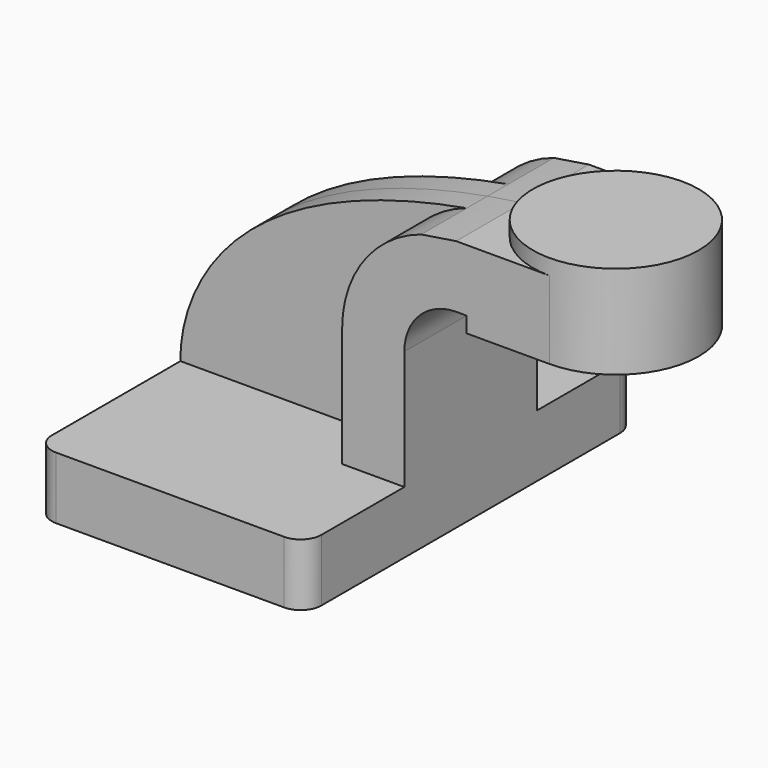
from build123d import *

# Parameters (mm, degrees)
F1_DEPTH = 63.5
F2_DEPTH = 25.4
F3_DEPTH = 7.9375
F5_R     = 6.35


# Not quite as in the source:
# - a feature names something its author has since deleted; it is built from what else it names


with BuildPart() as f1:
    # F0 (on Front) → F1 (new body, symmetric)
    with BuildSketch(Plane.XZ):
        Polygon((41.275, -9.525), (41.275, 9.525), (22.225, 9.525), (-41.275, 9.525), (-41.275, -9.525), align=None)
    extrude(amount=F1_DEPTH, both=True)

    # F0 (on Front) → F2 (join, symmetric)
    with BuildSketch(Plane.XZ):
        with BuildLine():
            Line((22.225, 9.525), (41.275, 9.525))
            Line((41.275, 9.525), (41.275, 46.0502))
            ThreePointArc((41.275, 46.0502), (45.9246798487, 57.2755201513), (57.15, 61.9252))
            Line((57.15, 61.9252), (60.325, 61.9252))
            Line((60.325, 61.9252), (60.325, 80.9752))
            Line((60.325, 80.9752), (57.15, 80.9752))
            add(Edge.make_bspline(
                [(46.42519144, 79.2877406183), (49.8648948299, 79.9027002695), (53.4381248944, 80.4666827005), (57.15, 80.9752)],
                knots=[116.6855453381, 116.6855453381, 116.6855453381, 116.6855453381, 121.6248811101, 121.6248811101, 121.6248811101, 121.6248811101], degree=3))
            ThreePointArc((46.42519144, 79.2877406183), (28.9159818308, 66.6073360608), (22.225, 46.0502))
            Line((22.225, 46.0502), (22.225, 9.525))
        make_face()
        Polygon((60.325, 80.9752), (60.325, 61.9252), (60.325, 57.15), (85.725, 57.15), (85.725, 80.9752), align=None)
    extrude(amount=F2_DEPTH, both=True)

    # F0 (on Front) → F3 (join, symmetric)
    with BuildSketch(Plane.XZ):
        with BuildLine():
            Line((-41.275, 9.525), (22.225, 9.525))
            Line((22.225, 9.525), (22.225, 46.0502))
            ThreePointArc((22.225, 46.0502), (28.9159818308, 66.6073360608), (46.42519144, 79.2877406183))
            add(Edge.make_bspline(
                [(-41.275, 9.525), (-41.5734088799, 21.7830526255), (-34.833440161, 64.760098527), (46.42519144, 79.2877406183)],
                knots=[0, 0, 0, 0, 116.6855453381, 116.6855453381, 116.6855453381, 116.6855453381], degree=3))
        make_face()
    extrude(amount=F3_DEPTH, both=True)

    # F0 (on Front) → F4 (revolve)
    with BuildSketch(Plane.XZ):
        Polygon((85.725, 80.9752), (85.725, 57.15), (111.125, 57.15), (111.125, 85.725), (85.725, 85.725), align=None)
    revolve(axis=Axis((85.725, 0, 71.4375), (0, 0, 1)))

    # F5
    f5_edges = [f1.edges().sort_by_distance(p)[0] for p in [
        (41.275, -63.5, 0),
        (-41.275, -63.5, 0),
        (-41.275, 63.5, 0),
        (41.275, 63.5, 0),
    ]]
    fillet(f5_edges, radius=F5_R)


solid = f1.part
